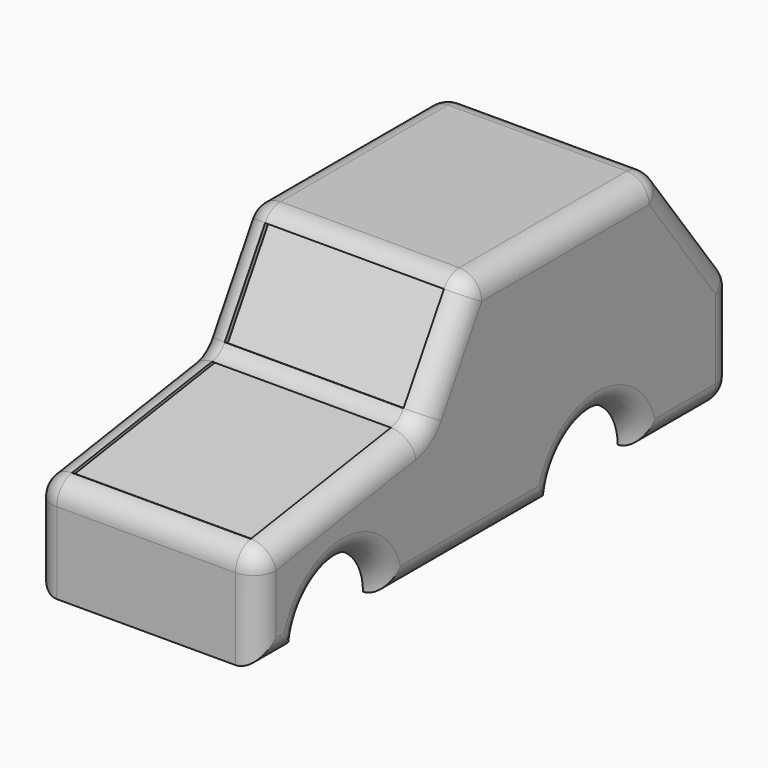
from build123d import *

# Parameters (mm, degrees)
F1_DEPTH = 25
F2_DEPTH = 25
F3_R     = 5
F4_T     = 2.5
F5_DEPTH = 1
F6_DEPTH = 1


# Not quite as in the source:
# - a shell that OpenCascade refuses in one call is made with other operations: the cavity is built on its own and cut out


with BuildPart() as f1:
    # F0 (on Right) → F1 (new body)
    with BuildSketch(Plane.YZ):
        with BuildLine():
            ThreePointArc((20.2099147212, 0), (32.2099147212, 12), (44.2099147212, 0))
            Line((44.2099147212, 0), (70.3801229509, 0))
            Line((70.3801229509, 0), (70.3801229509, 24.245692417))
            Line((70.3801229509, 24.245692417), (49.2672435939, 52.8463340897))
            Line((49.2672435939, 52.8463340897), (-2.9094794299, 52.8463340897))
            Line((-2.9094794299, 52.8463340897), (-16.8749988079, 29.4827595353))
            Line((-16.8749988079, 29.4827595353), (-62.6198770491, 22.5000027567))
            Line((-62.6198770491, 22.5000027567), (-62.6198770491, 0))
            Line((-62.6198770491, 0), (-51.0100852788, 0))
            ThreePointArc((-51.0100852788, 0), (-39.0100852788, 12), (-27.0100852788, 0))
            Line((-27.0100852788, 0), (20.2099147212, 0))
        make_face()
    extrude(amount=F1_DEPTH)

    # F2 (add): a face of the model
    f2_faces = [f1.faces().sort_by_distance(p)[0] for p in [
        (0, 12.6418380121, 23.4817334962),
    ]]
    extrude(f2_faces, amount=F2_DEPTH)

    # F3
    f3_edges = [f1.edges().sort_by_distance(p)[0] for p in [
        (0, 49.267244, 52.846334),
        (25, 70.380123, 12.122846),
        (25, -3.400085, 0),
        (25, 32.209915, 12),
        (25, 57.295019, 0),
        (25, 59.823683, 38.546013),
        (25, 23.178882, 52.846334),
        (25, -9.892239, 41.164547),
        (25, -39.747438, 25.991381),
        (25, -62.619877, 11.250001),
        (25, -56.814981, 0),
        (25, -39.010085, 12),
        (0, -62.619877, 22.500003),
        (-25, -39.747438, 25.991381),
        (0, -16.874999, 29.48276),
        (-25, -9.892239, 41.164547),
        (0, -2.909479, 52.846334),
        (-25, -3.400085, 0),
        (-25, 32.209915, 12),
        (-25, 57.295019, 0),
        (-25, 70.380123, 12.122846),
        (-25, 59.823683, 38.546013),
        (-25, 23.178882, 52.846334),
        (-25, -62.619877, 11.250001),
        (-25, -56.814981, 0),
        (-25, -39.010085, 12),
        (0, 70.380123, 24.245692),
        (0, 70.380123, 0),
    ]]
    fillet(f3_edges, radius=F3_R)

    # F4: shell of thickness 2.5, made by hand


with BuildPart() as f4_core1:
    # F4_t2: copy of F1
    add(f1.part)

    # the walls: a layer under each face that stays
    f4_faces = [f4_core1.faces().sort_by_distance(p)[0] for p in [
        (23.5355339059, -3.4000852788, 1.4644660941),
        (-23.5355339059, -3.4000852788, 1.4644660941),
        (23.5355339059, -39.0100852788, 13.4644660941),
        (-23.5355339059, -39.0100852788, 13.4644660941),
        (25, 3.8801229509, 26.4231670448),
        (23.5355339059, 32.2099147212, 13.4644660941),
        (-25, 3.8801229509, 26.4231670448),
        (-23.5355339059, 32.2099147212, 13.4644660941),
        (0, -62.6198770491, 9.1026573551),
        (23.5355339059, -56.8149811639, 1.4644660941),
        (-23.5355339077, -56.8149811639, 1.4644660958),
        (23.5355339059, 68.9156568568, 13.8000516084),
        (23.5355339059, 54.7950188361, 1.4644660941),
        (23.5355339059, 58.9062515794, 37.3229891204),
        (23.5355339059, 23.3352022927, 51.3818679956),
        (23.5355339059, -8.7585703239, 40.2068135939),
        (23.5355339059, -16.3521210361, 28.7047847532),
        (23.5355339059, -38.5680150875, 24.689985527),
        (23.5355339059, -61.155410955, 9.1026573551),
        (-23.5355339059, -38.5680150875, 24.689985527),
        (-23.5355339059, -16.3521210361, 28.7047847532),
        (-23.5355339059, -61.155410955, 9.1026573551),
        (-23.5355339059, -8.7585703239, 40.2068135939),
        (-23.5355339059, 23.3352022927, 51.3818679956),
        (-23.5355339059, 58.9062515794, 37.3229891204),
        (-23.5355339059, 68.9156568568, 13.8000516084),
        (-23.5355339059, 54.7950188361, 1.4644660941),
        (0, 68.9156568568, 1.4644660941),
        (0, -61.4127944026, 21.4631940741),
        (0, 70.3801229509, 13.8000516084),
        (22.5, 67.8801229509, 1.4644660941),
        (23.5355339059, 68.7384478155, 23.7053878424),
        (0, 60.0844663113, 38.1927425258),
        (23.5355339059, 48.3365962689, 51.0025826288),
        (0, 23.3352022927, 52.8463340897),
        (23.5355339059, -1.8175547252, 50.9215103494),
        (0, -10.0155870481, 40.9581922572),
        (0, -17.1690279113, 29.9202369726),
        (0, -38.7889997465, 26.1376825675),
        (23.5355339059, -60.3018746302, 20.5089833007),
        (-23.5355339059, -60.3018746302, 20.5089833007),
        (-23.5355339059, -1.8175547252, 50.9215103494),
        (-23.5355339059, 48.3365962689, 51.0025826288),
        (-23.5355339059, 68.7384478155, 23.7053878424),
        (-22.5, 68.9156568568, 2.5),
        (0, 70.1295115213, 24.1632117246),
        (0, 48.9964964766, 52.3099435799),
        (0, -2.5401515576, 52.1952900629),
    ]]
    thicken(f4_faces, amount=-F4_T, mode=Mode.SUBTRACT)


with BuildPart() as f1_1:
    add(f1.part)

    # what is left inside the walls is the cavity
    f4_cavity = [f4_core1.part.solids().sort_by_distance(p)[0] for p in [
        (-22.475, 3.880123, 19.282111),
    ]]
    add(f4_cavity, mode=Mode.SUBTRACT)

    # F5 (cut): faces of the model
    f5_faces = [f1_1.faces().sort_by_distance(p)[0] for p in [
        (0, -10.0155870481, 40.9581922572),
        (0, -38.7889997465, 26.1376825675),
    ]]
    extrude(f5_faces, amount=-F5_DEPTH, dir=(0, -0.8583447096, 0.5130734446), mode=Mode.SUBTRACT)

    # F6 (cut): faces of the model
    f6_faces = [f1_1.faces().sort_by_distance(p)[0] for p in [
        (0, 70.3801229509, 13.8000516084),
        (0, 60.0844663113, 38.1927425258),
    ]]
    extrude(f6_faces, amount=-F6_DEPTH, dir=(0, 1, 0), mode=Mode.SUBTRACT)


solid = f1_1.part
